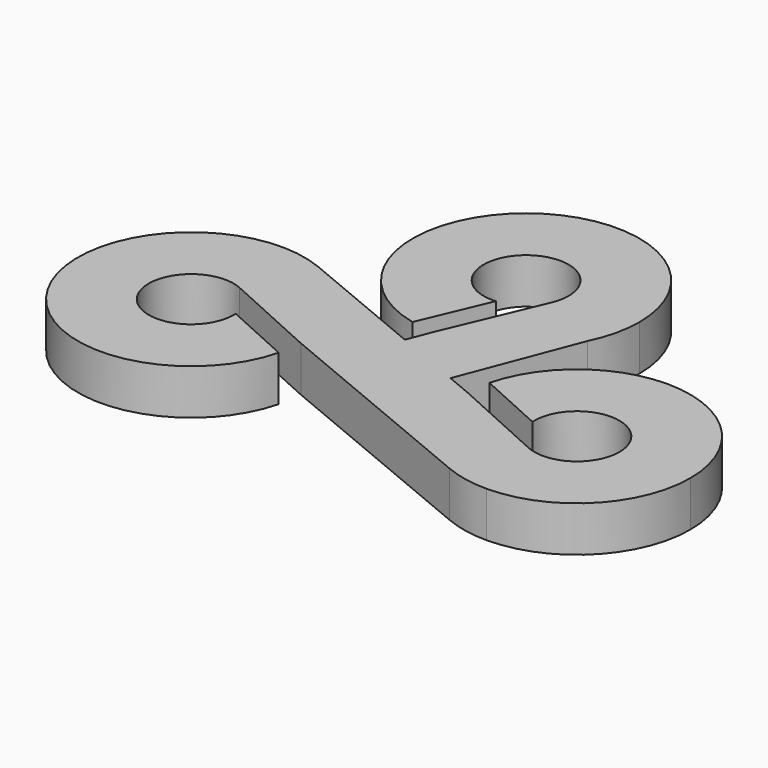
from build123d import *

# Parameters (mm, degrees)
F1_DEPTH = 5.08
F3_DEPTH = 25.4


# Not quite as in the source:
# - a feature names something its author has since deleted; it is built from what else it names


with BuildPart() as f1:
    # F0 (on Top) → F1 (new body)
    with BuildSketch(Plane.XY):
        with BuildLine():
            Line((6.7351920908, -6.7351920908), (8.9802561211, -8.9802561211))
            ThreePointArc((8.9802561211, -8.9802561211), (10.3222667059, -7.3987032683), (11.3889377966, -5.619795002))
            ThreePointArc((11.3889377966, -5.619795002), (12.3678921005, -2.8853500639), (12.7, 0))
            ThreePointArc((12.7, 0), (-8.9094308211, 9.0505271915), (-0.1995342432, -12.6984324263))
            Line((-0.1995342432, -12.6984324263), (0, -12.1764942784))
            Line((0, -12.1764942784), (0, -4.7625))
            ThreePointArc((0, -4.7625), (-3.3675960454, 3.3675960454), (4.7625, 0))
            ThreePointArc((4.7625, 0), (4.3999762736, -1.8225298466), (3.3675960454, -3.3675960454))
            Line((3.3675960454, -3.3675960454), (4.4901280605, -4.4901280605))
            Line((4.4901280605, -4.4901280605), (6.7351920908, -6.7351920908))
        make_face()
        with BuildLine():
            ThreePointArc((11.3889377966, -5.619795002), (10.3222667059, -7.3987032683), (8.9802561211, -8.9802561211))
            ThreePointArc((8.9802561211, -8.9802561211), (6.8924812287, -10.6669443849), (4.4968663349, -11.8772131902))
            Line((4.4968663349, -11.8772131902), (2.3084511304, -16.9045766677))
            Line((2.3084511304, -16.9045766677), (6.4203654177, -18.6164988404))
            Line((6.4203654177, -18.6164988404), (11.3889377966, -5.619795002))
        make_face()
        with BuildLine():
            Line((2.3084511304, -16.9045766677), (4.4968663349, -11.8772131902))
            ThreePointArc((4.4968663349, -11.8772131902), (2.2857594454, -12.4926099658), (0, -12.7))
            ThreePointArc((0, -12.7), (-0.0997702004, -12.6996081005), (-0.1995342432, -12.6984324263))
            Line((-0.1995342432, -12.6984324263), (-1.2423673122, -15.4262567422))
            Line((-1.2423673122, -15.4262567422), (2.3084511304, -16.9045766677))
        make_face()
        with BuildLine():
            Line((9.2538210972, -19.7961575745), (6.4203654177, -18.6164988404))
            Line((6.4203654177, -18.6164988404), (2.3084511304, -16.9045766677))
            Line((2.3084511304, -16.9045766677), (0.652517293, -20.7086908404))
            Line((0.652517293, -20.7086908404), (10.0662240577, -24.8064846655))
            ThreePointArc((10.0662240577, -24.8064846655), (9.4071650605, -22.3423208774), (9.2538210972, -19.7961575745))
        make_face()
        with BuildLine():
            ThreePointArc((-0.1995342432, -12.6984324263), (-0.0997702004, -12.6996081005), (0, -12.7))
            Line((0, -12.7), (0, -12.1764942784))
            Line((0, -12.1764942784), (-0.1995342432, -12.6984324263))
        make_face()
        with BuildLine():
            Line((0.652517293, -20.7086908404), (2.3084511304, -16.9045766677))
            Line((2.3084511304, -16.9045766677), (-1.2423673122, -15.4262567422))
            Line((-1.2423673122, -15.4262567422), (-15.757129186, -9.3832945241))
            ThreePointArc((-15.757129186, -9.3832945241), (-13.5731230118, -10.5544783892), (-11.6581465409, -12.1275072291))
            ThreePointArc((-11.6581465409, -12.1275072291), (-9.971458277, -14.2152821214), (-8.7611894717, -16.6108970152))
            Line((-8.7611894717, -16.6108970152), (0.652517293, -20.7086908404))
        make_face()
        with BuildLine():
            Line((18.5758412025, -23.677214376), (9.2538210972, -19.7961575745))
            ThreePointArc((9.2538210972, -19.7961575745), (9.4071650605, -22.3423208774), (10.0662240577, -24.8064846655))
            Line((10.0662240577, -24.8064846655), (15.2082451571, -27.0448104214))
            Line((15.2082451571, -27.0448104214), (17.4533091874, -24.7997463911))
            Line((17.4533091874, -24.7997463911), (18.5758412025, -23.677214376))
        make_face()
        with BuildLine():
            ThreePointArc((34.6434372479, -20.3096183306), (22.2002201194, -7.6122145583), (9.2538210972, -19.7961575745))
            Line((9.2538210972, -19.7961575745), (18.5758412025, -23.677214376))
            ThreePointArc((18.5758412025, -23.677214376), (20.1209074013, -15.909642057), (26.7059372479, -20.3096183306))
            ThreePointArc((26.7059372479, -20.3096183306), (25.3110332933, -23.677214376), (21.9434372479, -25.0721183306))
            Line((21.9434372479, -25.0721183306), (21.9434372479, -33.0096183306))
            ThreePointArc((21.9434372479, -33.0096183306), (30.923693369, -29.2898744517), (34.6434372479, -20.3096183306))
        make_face()
        with BuildLine():
            Line((10.0662240577, -24.8064846655), (0.652517293, -20.7086908404))
            Line((0.652517293, -20.7086908404), (-8.7611894717, -16.6108970152))
            ThreePointArc((-8.7611894717, -16.6108970152), (-8.1457926961, -18.8220039048), (-7.9384026619, -21.1077633501))
            ThreePointArc((-7.9384026619, -21.1077633501), (-7.9409988896, -21.3645462216), (-7.9487865112, -21.6212241063))
            Line((-7.9487865112, -21.6212241063), (17.062163772, -32.0340871567))
            ThreePointArc((17.062163772, -32.0340871567), (14.8781575978, -30.8629032915), (12.9631811269, -29.2898744517))
            ThreePointArc((12.9631811269, -29.2898744517), (11.276492863, -27.2020995593), (10.0662240577, -24.8064846655))
        make_face()
        with BuildLine():
            ThreePointArc((21.9434372479, -25.0721183306), (20.1209074013, -24.7095946042), (18.5758412025, -23.677214376))
            Line((18.5758412025, -23.677214376), (17.4533091874, -24.7997463911))
            Line((17.4533091874, -24.7997463911), (15.2082451571, -27.0448104214))
            Line((15.2082451571, -27.0448104214), (12.9631811269, -29.2898744517))
            ThreePointArc((12.9631811269, -29.2898744517), (14.8781575978, -30.8629032915), (17.062163772, -32.0340871567))
            ThreePointArc((17.062163772, -32.0340871567), (19.4545372993, -32.7633477739), (21.9434372479, -33.0096183306))
            Line((21.9434372479, -33.0096183306), (21.9434372479, -25.0721183306))
        make_face()
        with BuildLine():
            ThreePointArc((-11.6581465409, -12.1275072291), (-13.5731230118, -10.5544783892), (-15.757129186, -9.3832945241))
            ThreePointArc((-15.757129186, -9.3832945241), (-31.3447452065, -27.9388854628), (-7.9487865112, -21.6212241063))
            Line((-7.9487865112, -21.6212241063), (-9.1820824244, -21.1077633501))
            Line((-9.1820824244, -21.1077633501), (-15.8759026619, -21.1077633501))
            ThreePointArc((-15.8759026619, -21.1077633501), (-25.0383789355, -22.9302931968), (-17.2708066165, -17.7401673047))
            Line((-17.2708066165, -17.7401673047), (-16.1482746014, -16.6176352896))
            Line((-16.1482746014, -16.6176352896), (-13.9032105711, -14.3725712593))
            Line((-13.9032105711, -14.3725712593), (-11.6581465409, -12.1275072291))
        make_face()
        with BuildLine():
            Line((-9.1820824244, -21.1077633501), (-7.9487865112, -21.6212241063))
            ThreePointArc((-7.9487865112, -21.6212241063), (-7.9409988896, -21.3645462216), (-7.9384026619, -21.1077633501))
            Line((-7.9384026619, -21.1077633501), (-9.1820824244, -21.1077633501))
        make_face()
        with BuildLine():
            Line((15.2082451571, -27.0448104214), (10.0662240577, -24.8064846655))
            ThreePointArc((10.0662240577, -24.8064846655), (11.276492863, -27.2020995593), (12.9631811269, -29.2898744517))
            Line((12.9631811269, -29.2898744517), (15.2082451571, -27.0448104214))
        make_face()
        with BuildLine():
            ThreePointArc((0, -12.7), (2.2857594454, -12.4926099658), (4.4968663349, -11.8772131902))
            Line((4.4968663349, -11.8772131902), (6.7351920908, -6.7351920908))
            Line((6.7351920908, -6.7351920908), (4.4901280605, -4.4901280605))
            Line((4.4901280605, -4.4901280605), (3.3675960454, -3.3675960454))
            Line((3.3675960454, -3.3675960454), (0, -12.1764942784))
            Line((0, -12.1764942784), (0, -12.7))
        make_face()
        with BuildLine():
            Line((-15.8759026619, -21.1077633501), (-9.1820824244, -21.1077633501))
            Line((-9.1820824244, -21.1077633501), (-17.2708066165, -17.7401673047))
            ThreePointArc((-17.2708066165, -17.7401673047), (-16.2384263884, -19.2852335035), (-15.8759026619, -21.1077633501))
        make_face()
        with BuildLine():
            ThreePointArc((-7.9384026619, -21.1077633501), (-8.1457926961, -18.8220039048), (-8.7611894717, -16.6108970152))
            Line((-8.7611894717, -16.6108970152), (-13.9032105711, -14.3725712593))
            Line((-13.9032105711, -14.3725712593), (-16.1482746014, -16.6176352896))
            Line((-16.1482746014, -16.6176352896), (-17.2708066165, -17.7401673047))
            Line((-17.2708066165, -17.7401673047), (-9.1820824244, -21.1077633501))
            Line((-9.1820824244, -21.1077633501), (-7.9384026619, -21.1077633501))
        make_face()
        with BuildLine():
            Line((0, -4.7625), (0, -12.1764942784))
            Line((0, -12.1764942784), (3.3675960454, -3.3675960454))
            ThreePointArc((3.3675960454, -3.3675960454), (1.8225298466, -4.3999762736), (0, -4.7625))
        make_face()
        with BuildLine():
            Line((-13.9032105711, -14.3725712593), (-8.7611894717, -16.6108970152))
            ThreePointArc((-8.7611894717, -16.6108970152), (-9.971458277, -14.2152821214), (-11.6581465409, -12.1275072291))
            Line((-11.6581465409, -12.1275072291), (-13.9032105711, -14.3725712593))
        make_face()
        with BuildLine():
            ThreePointArc((4.4968663349, -11.8772131902), (6.8924812287, -10.6669443849), (8.9802561211, -8.9802561211))
            Line((8.9802561211, -8.9802561211), (6.7351920908, -6.7351920908))
            Line((6.7351920908, -6.7351920908), (4.4968663349, -11.8772131902))
        make_face()
    extrude(amount=F1_DEPTH)

    # F2 (on face) → F3 (cut)
    with BuildSketch(Plane.XY.offset(5.08)):
        with BuildLine():
            Line((-15.8846679825, -20.8189505253), (-8.3298662663, -24.2366500209))
            ThreePointArc((-8.3298662663, -24.2366500209), (-8.0711029973, -22.9388775299), (-7.9487865112, -21.6212241063))
            Line((-7.9487865112, -21.6212241063), (-18.6754288181, -16.7686228893))
            ThreePointArc((-18.6754288181, -16.7686228893), (-16.7166897918, -18.4056207903), (-15.8846679825, -20.8189505253))
        make_face()
        with BuildLine():
            ThreePointArc((-2.823583262, -12.3821394582), (-1.5198092555, -12.6087342674), (-0.1995342432, -12.6984324263))
            Line((-0.1995342432, -12.6984324263), (4.3863512165, -1.8550820077))
            ThreePointArc((4.3863512165, -1.8550820077), (2.7982865403, -3.8536993511), (0.406267641, -4.7451399193))
            Line((0.406267641, -4.7451399193), (-2.823583262, -12.3821394582))
        make_face()
        with BuildLine():
            ThreePointArc((9.6349008523, -17.1807316599), (9.3761375833, -18.4785041508), (9.2538210972, -19.7961575745))
            Line((9.2538210972, -19.7961575745), (19.9804634041, -24.6487587914))
            ThreePointArc((19.9804634041, -24.6487587914), (18.0217243778, -23.0117608905), (17.1897025685, -20.5984311555))
            Line((17.1897025685, -20.5984311555), (9.6349008523, -17.1807316599))
        make_face()
    extrude(amount=-F3_DEPTH, mode=Mode.SUBTRACT)


solid = f1.part
